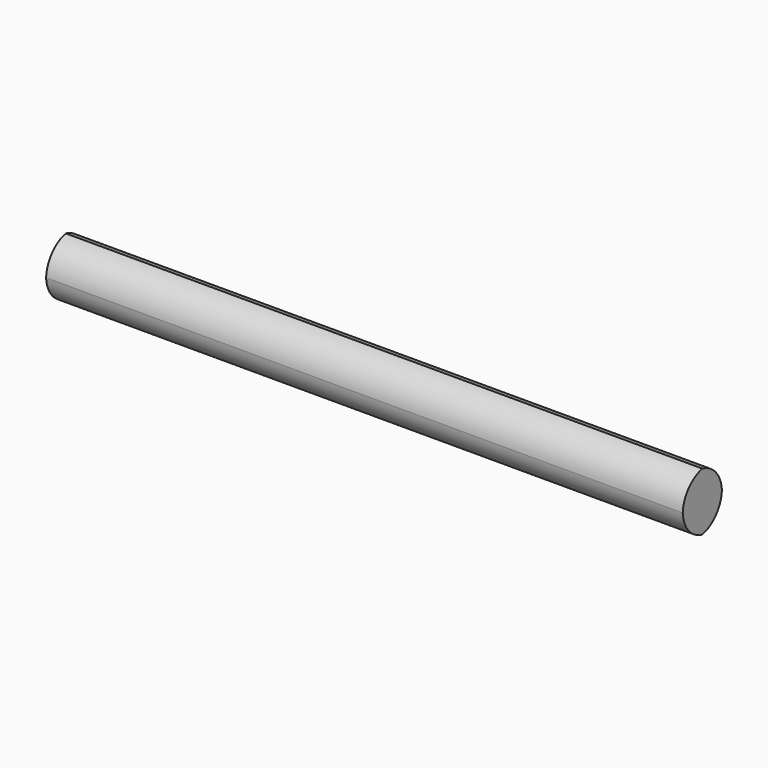
from build123d import *

# Parameters (mm, degrees)
F0_W        = 7.8271683306
F0_H        = 9.5099005848
F2_DEPTH    = 25
F3_DEPTH    = 25
F1_W        = 7.8271683306
F1_H        = 9.5099005848
F4_DEPTH    = 51.5792816877
F3_FACE_W   = 7.8271683306
F3_FACE_H   = 9.5099005848
F4_FACE_W   = 7.8271683306
F4_FACE_H   = 9.5099005848
F6_T1_DEPTH = 126.5792816877


# Not quite as in the source:
# - a fillet or chamfer that OpenCascade refuses, or shapes differently, is made with other operations: its cross-section is extruded or revolved along the edge and cut away or added


with BuildPart() as f2:
    # F0 (on Right) → F2 (new body)
    with BuildSketch(Plane.YZ):
        with Locations((-22.5047236308, 34.8080685362)):
            Rectangle(F0_W, F0_H)
    extrude(amount=F2_DEPTH)

    # F3 (add): a face of the model
    f3_faces = [f2.faces().sort_by_distance(p)[0] for p in [
        (25, -22.5047236308, 34.8080685362),
    ]]
    extrude(f3_faces, amount=F3_DEPTH)

    # F1 (on face) → F4 (join)
    with BuildSketch(Plane.YZ):
        with Locations((-22.5047236308, 34.8080685362)):
            Rectangle(F1_W, F1_H)
    extrude(amount=-F4_DEPTH)

    # F3_face (on face) → F5 section 0
    with BuildSketch(Plane(origin=(50, -22.5047236308, 34.8080685362), x_dir=(0, 1, 0), z_dir=(1, 0, 0))):
        Rectangle(F3_FACE_W, F3_FACE_H)
    # F4_face (on face) → F5 section 1
    with BuildSketch(Plane(origin=(-51.5792816877, -22.5047236308, 34.8080685362), x_dir=(0, 1, 0), z_dir=(-1, 0, 0))):
        Rectangle(F4_FACE_W, F4_FACE_H)
    loft()

    # F6: fillet of radius 5 on 4 edges, made by hand

    # F6_s2 → F6_t1 (cut)
    with BuildSketch(Plane.YZ.offset(-64.0792816877)):
        with BuildLine():
            ThreePointArc((-21.4183077961, 39.5630188286), (-24.9538417021, 38.0985527346), (-26.4183077961, 34.5630188286))
            Line((-26.4183077961, 34.5630188286), (-26.4183077961, 39.5630188286))
            Line((-26.4183077961, 39.5630188286), (-21.4183077961, 39.5630188286))
        make_face()
        with BuildLine():
            ThreePointArc((-23.5911394656, 39.5630188286), (-20.0556055596, 38.0985527346), (-18.5911394656, 34.5630188286))
            Line((-18.5911394656, 34.5630188286), (-18.5911394656, 39.5630188286))
            Line((-18.5911394656, 39.5630188286), (-23.5911394656, 39.5630188286))
        make_face()
        with BuildLine():
            ThreePointArc((-26.4183077961, 35.0531182438), (-24.9538417021, 31.5175843379), (-21.4183077961, 30.0531182438))
            Line((-21.4183077961, 30.0531182438), (-26.4183077961, 30.0531182438))
            Line((-26.4183077961, 30.0531182438), (-26.4183077961, 35.0531182438))
        make_face()
        with BuildLine():
            ThreePointArc((-18.5911394656, 35.0531182438), (-20.0556055596, 31.5175843379), (-23.5911394656, 30.0531182438))
            Line((-23.5911394656, 30.0531182438), (-18.5911394656, 30.0531182438))
            Line((-18.5911394656, 30.0531182438), (-18.5911394656, 35.0531182438))
        make_face()
    extrude(amount=F6_T1_DEPTH, mode=Mode.SUBTRACT)


solid = f2.part
